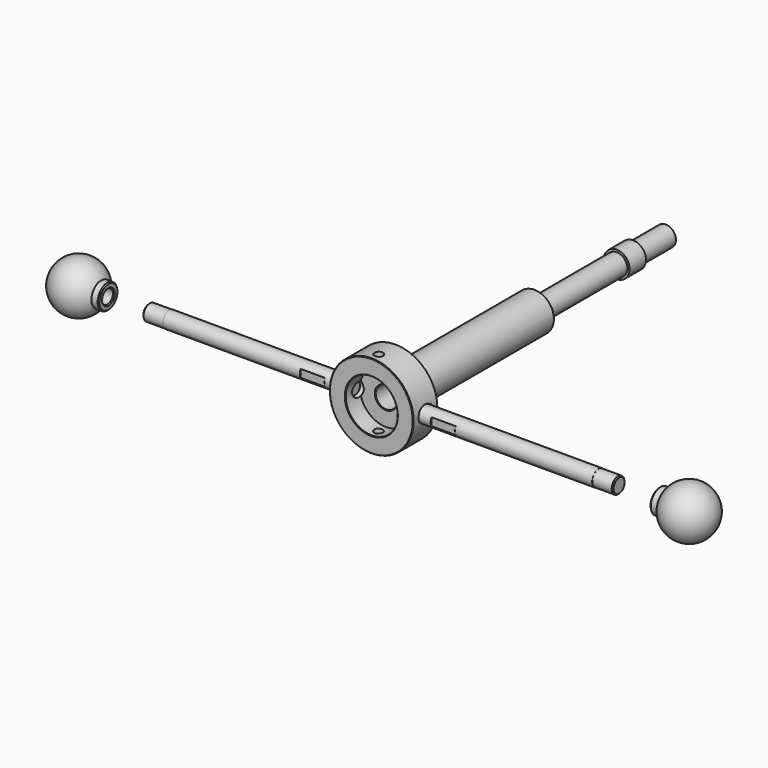
from build123d import *

# Parameters (mm, degrees)
F0_R      = 20.5
F1_DEPTH  = 15
F2_R      = 9.5
F3_DEPTH  = 85
F4_R      = 12.725
F5_DEPTH  = 9
F6_R      = 5.25
F7_DEPTH  = 91.001
F8_SIZE   = 0.25
F10_R     = 4.5
F11_DEPTH = 0.5
F13_D     = 6.8
F13_DEPTH = 8
F13_TIP   = 2.0429261047
F15_R     = 4.5
F16_DEPTH = 0.5
F18_D     = 6.8
F18_DEPTH = 8
F18_TIP   = 2.0429261047
F19_R     = 3.4
F20_DEPTH = 6
F21_R     = 3.9900235839
F22_DEPTH = 85
F23_R     = 3.9
F24_DEPTH = 10
F25_SIZE  = 0.5
F30_R     = 3.4
F31_DEPTH = 15
F32_SIZE  = 0.5
F35_W     = 12
F35_H     = 9
F36_DEPTH = 0.5
F37_W     = 12
F37_H     = 3.8315992485
F38_DEPTH = 0.5
F40_R     = 2.1
F41_DEPTH = 25
F42_R     = 5.25
F43_DEPTH = 50
F44_R     = 6.35
F45_DEPTH = 10
F46_R     = 5
F47_DEPTH = 20


with BuildPart() as f1:
    # F0 (on Front) → F1 (new body)
    with BuildSketch(Plane.XZ):
        Circle(F0_R)
    extrude(amount=-F1_DEPTH)

    # F2 (on face) → F3 (join)
    with BuildSketch(Plane(origin=(0, 15, 0), x_dir=(-1, 0, 0), z_dir=(0, 1, 0))):
        Circle(F2_R)
    extrude(amount=F3_DEPTH)

    # F4 (on face) → F5 (cut)
    with BuildSketch(Plane.XZ):
        Circle(F4_R)
    extrude(amount=-F5_DEPTH, mode=Mode.SUBTRACT)

    # F6 (on face) → F7 (cut, through all)
    with BuildSketch(Plane.XZ.offset(-9)):
        Circle(F6_R)
    extrude(amount=-F7_DEPTH, mode=Mode.SUBTRACT)

    # F8
    f8_edges = [f1.edges().sort_by_distance(p)[0] for p in [
        (-20.5, 0, 0),
        (-12.725, 0, 0),
        (-5.25, 9, 0),
        (5.25, 54.5, 0),
        (-5.25, 100, 0),
        (20.5, 7.5, 0),
        (-20.5, 15, 0),
        (9.5, 100, 0),
    ]]
    chamfer(f8_edges, length=F8_SIZE)

    # F10 (on offset) → F11 (cut)
    with BuildSketch(Plane.YZ.offset(20.5)):
        with Locations((7.75, 0)):
            Circle(F10_R)
    extrude(amount=-F11_DEPTH, mode=Mode.SUBTRACT)

    # F13
    with Locations(Plane.YZ.offset(20)):
        with Locations((7.75, 0)):
            Hole(F13_D / 2, depth=F13_DEPTH)
            with Locations((0, 0, -(F13_DEPTH + F13_TIP / 2))):  # 118° drill point
                Cone(0, F13_D / 2, F13_TIP, mode=Mode.SUBTRACT)

    # F15 (on offset) → F16 (cut)
    with BuildSketch(Plane.YZ.offset(-20.5)):
        with Locations((7.5, 0)):
            Circle(F15_R)
    extrude(amount=F16_DEPTH, mode=Mode.SUBTRACT)

    # F18
    with Locations(Plane(origin=(-20, 0, 0), x_dir=(0, -1, 0), z_dir=(-1, 0, 0))):
        with Locations((-7.5, 0)):
            Hole(F18_D / 2, depth=F18_DEPTH)
            with Locations((0, 0, -(F18_DEPTH + F18_TIP / 2))):  # 118° drill point
                Cone(0, F18_D / 2, F18_TIP, mode=Mode.SUBTRACT)

    # F40 (on Top) → F41 (cut, symmetric)
    with BuildSketch(Plane.XY):
        with Locations((0, 4.5)):
            Circle(F40_R)
    extrude(amount=F41_DEPTH, both=True, mode=Mode.SUBTRACT)


with BuildPart() as f20:
    # F19 (on face) → F20 (new body)
    with BuildSketch(Plane.YZ.offset(20)):
        with Locations((7.75, 0)):
            Circle(F19_R)
    extrude(amount=-F20_DEPTH)

    # F21 (on face) → F22 (join)
    with BuildSketch(Plane.YZ.offset(20)):
        with Locations((7.75, 0)):
            Circle(F21_R)
    extrude(amount=F22_DEPTH)

    # F23 (on face) → F24 (join)
    with BuildSketch(Plane.YZ.offset(105)):
        with Locations((7.75, 0)):
            Circle(F23_R)
    extrude(amount=F24_DEPTH)

    # F25
    f25_edges = [f20.edges().sort_by_distance(p)[0] for p in [
        (14, 4.35, 0),
        (115, 3.85, 0),
    ]]
    chamfer(f25_edges, length=F25_SIZE)

    # F35 (on offset) → F36 (cut)
    with BuildSketch(Plane.XZ.offset(-3.75)):
        with Locations((32, 0)):
            Rectangle(F35_W, F35_H)
    extrude(amount=-F36_DEPTH, mode=Mode.SUBTRACT)

    # F37 (on offset) → F38 (cut)
    with BuildSketch(Plane.XZ.offset(-11.75)):
        with Locations((32, 0)):
            Rectangle(F37_W, F37_H)
    extrude(amount=F38_DEPTH, mode=Mode.SUBTRACT)


with BuildPart() as f29:
    # F28 (on plane+point) → F29 (revolve)
    with BuildSketch(Plane.XZ.offset(-7.75)):
        with BuildLine():
            Line((134.7739224189, 0), (161.7739224189, 0))
            ThreePointArc((161.7739224189, 0), (152.3704364875, 12.1103922572), (138.3080663192, 6))
            Line((138.3080663192, 6), (134.7739224189, 6))
            Line((134.7739224189, 6), (134.7739224189, 0))
        make_face()
    revolve(axis=Axis((148.2739224189, 7.75, 0), (1, 0, 0)))

    # F30 (on face) → F31 (cut)
    with BuildSketch(Plane(origin=(134.7739224189, 0, 0), x_dir=(0, -1, 0), z_dir=(-1, 0, 0))):
        with Locations((-7.75, 0)):
            Circle(F30_R)
    extrude(amount=-F31_DEPTH, mode=Mode.SUBTRACT)

    # F32
    f32_edges = [f29.edges().sort_by_distance(p)[0] for p in [
        (134.773922, 7.75, -6),
        (134.773922, 11.15, 0),
    ]]
    chamfer(f32_edges, length=F32_SIZE)


with BuildPart() as f39_1:
    # F39: instance of F20
    add(f20.part.mirror(Plane.YZ))


with BuildPart() as f39_2:
    # F39: instance of F29
    add(f29.part.mirror(Plane.YZ))


with BuildPart() as f43:
    # F42 (on face) → F43 (new body)
    with BuildSketch(Plane(origin=(0, 100, 0), x_dir=(-1, 0, 0), z_dir=(0, 1, 0))):
        Circle(F42_R)
    extrude(amount=F43_DEPTH)

    # F44 (on face) → F45 (join)
    with BuildSketch(Plane(origin=(0, 150, 0), x_dir=(-1, 0, 0), z_dir=(0, 1, 0))):
        Circle(F44_R)
    extrude(amount=F45_DEPTH)

    # F46 (on face) → F47 (join)
    with BuildSketch(Plane(origin=(0, 160, 0), x_dir=(-1, 0, 0), z_dir=(0, 1, 0))):
        Circle(F46_R)
    extrude(amount=F47_DEPTH)


solid = Compound([f1.part, f20.part, f29.part, f39_1.part, f39_2.part, f43.part])
